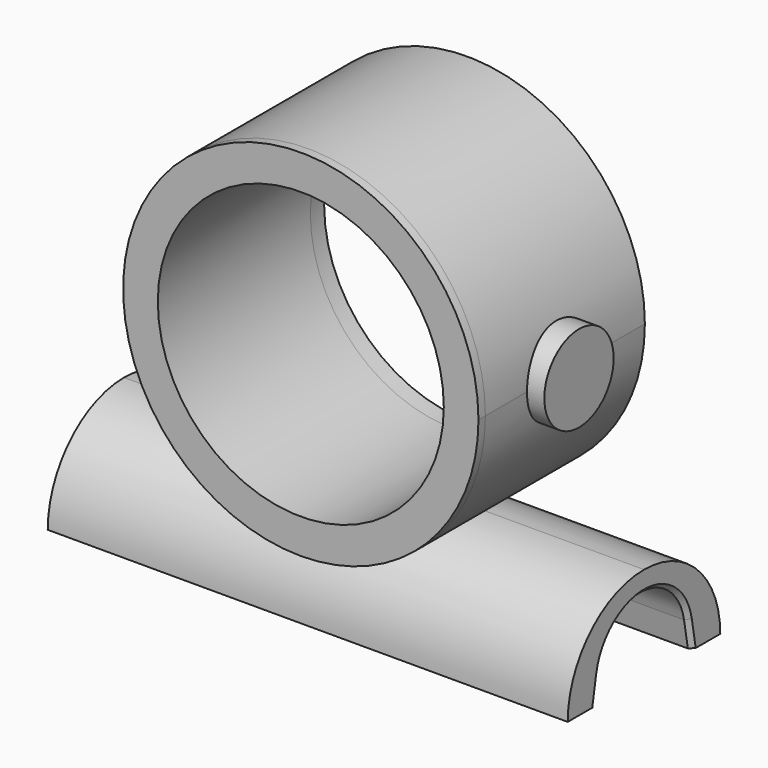
from build123d import *
from build123d import SkipClean  # not in build123d's __all__

# Parameters (mm, degrees)
F0_W            = 190.5
F0_H            = 69.85
F1_DEPTH        = 34.925
F4_DEPTH        = 190.5
F5_DEPTH        = 73.025
F6_DEPTH        = 3.175
F9_DEPTH        = 190.5010001
F10_SIZE2       = 1.5875
F10_SIZE        = 1.5875
F14_DEPTH       = 36.64824
F16_DEPTH       = 83.54939
F17_D           = 104.775
F17_CBORE_D     = 104.8004
F17_CBORE_DEPTH = 6.35


with BuildPart() as f1:
    # F0 (on Top) → F1 (new body)
    with BuildSketch(Plane.XY):
        Rectangle(F0_W, F0_H)
    extrude(amount=F1_DEPTH)

    # F2 (on face) → F4 (cut)
    with BuildSketch(Plane.YZ.offset(95.25)):
        with BuildLine():
            Line((-34.925, 34.925), (-34.925, 0))
            ThreePointArc((-34.925, 0), (-24.6957043451, 24.6957043208), (-3.45e-08, 34.925))
            Line((-3.45e-08, 34.925), (-34.925, 34.925))
        make_face()
        with BuildLine():
            ThreePointArc((-3.45e-08, 34.925), (24.6957043208, 24.6957043451), (34.925, 0))
            Line((34.925, 0), (34.925, 34.925))
            Line((34.925, 34.925), (-3.45e-08, 34.925))
        make_face()
    extrude(amount=-F4_DEPTH, mode=Mode.SUBTRACT)

    # F3 (on face) → F5 (join)
    with BuildSketch(Plane.XZ.offset(34.925)):
        with BuildLine():
            Line((-36.3741945787, 34.925), (0, 34.925))
            Line((0, 34.925), (36.3741945787, 34.925))
            ThreePointArc((36.3741945787, 34.925), (57.462544522, 58.3314110024), (65.0875, 88.9))
            ThreePointArc((65.0875, 88.9), (-30.5685889976, 146.362544522), (-36.3741945787, 34.925))
        make_face()
        with BuildLine():
            Line((0, 34.925), (0, 23.8125))
            ThreePointArc((0, 23.8125), (19.0168983243, 26.6525885327), (36.3741945787, 34.925))
            Line((36.3741945787, 34.925), (0, 34.925))
        make_face()
        with BuildLine():
            ThreePointArc((-36.3741945787, 34.925), (-19.0168983243, 26.6525885327), (0, 23.8125))
            Line((0, 23.8125), (0, 34.925))
            Line((0, 34.925), (-36.3741945787, 34.925))
        make_face()
    with SkipClean():  # cleaning this boolean's faces spoils the solid; the shape is the same uncleaned
        extrude(amount=-F5_DEPTH)

    # F6 (add): a face of the model
    f6_faces = [f1.faces().sort_by_distance(p)[0] for p in [
        (0, -34.925, 88.9),
    ]]
    with SkipClean():  # cleaning this boolean's faces spoils the solid; the shape is the same uncleaned
        extrude(f6_faces, amount=F6_DEPTH)

    # F8 (on face) → F9 (cut, through all)
    with BuildSketch(Plane.YZ.offset(95.25)):
        with BuildLine():
            Line((22.0755430303, 0), (20.3239700028, 9.9336642666))
            ThreePointArc((20.3239700028, 9.9336642666), (0, 26.9875), (-20.3239700028, 9.9336642666))
            Line((-20.3239700028, 9.9336642666), (-22.0755430303, 0))
            Line((-22.0755430303, 0), (0, 0))
            Line((0, 0), (22.0755430303, 0))
        make_face()
    with SkipClean():  # cleaning this boolean's faces spoils the solid; the shape is the same uncleaned
        extrude(amount=-F9_DEPTH, mode=Mode.SUBTRACT)

    # F10
    f10_edges = [f1.edges().sort_by_distance(p)[0] for p in [
        (95.25, 0, 26.9875),
        (95.25, 21.199757, 4.966832),
        (95.25, -21.199757, 4.966832),
        (-95.25, 0, 26.9875),
        (-95.25, -21.199757, 4.966832),
        (-95.25, 21.199757, 4.966832),
    ]]
    chamfer(f10_edges, length=F10_SIZE, length2=F10_SIZE2)

    # F13 (on face) → F14 (join)
    with BuildSketch(Plane.YZ.offset(95.25)):
        with BuildLine():
            ThreePointArc((15.875, 88.9), (-11.2253201513, 100.1253201513), (0, 73.025))
            ThreePointArc((0, 73.025), (11.2253201513, 77.6746798487), (15.875, 88.9))
        make_face()
    with SkipClean():  # cleaning this boolean's faces spoils the solid; the shape is the same uncleaned
        extrude(amount=-F14_DEPTH)

    # F15 (on face) → F16 (cut)
    with BuildSketch(Plane.XZ.offset(38.1)):
        Polygon((71.4375, 107.923515141), (71.4375, 88.9), (71.4375, 69.2154169083), (71.4375, 68.7513798475), (104.9063950777, 68.7513798475), (104.9063950777, 107.923515141), align=None)
    with SkipClean():  # cleaning this boolean's faces spoils the solid; the shape is the same uncleaned
        extrude(amount=-F16_DEPTH, mode=Mode.SUBTRACT)

    # F17 (through all)
    with Locations(Plane(origin=(0, 38.1, 0), x_dir=(-1, 0, 0), z_dir=(0, 1, 0))):
        with Locations((0, 88.9)):
            CounterBoreHole(F17_D / 2, F17_CBORE_D / 2, F17_CBORE_DEPTH)


solid = f1.part
